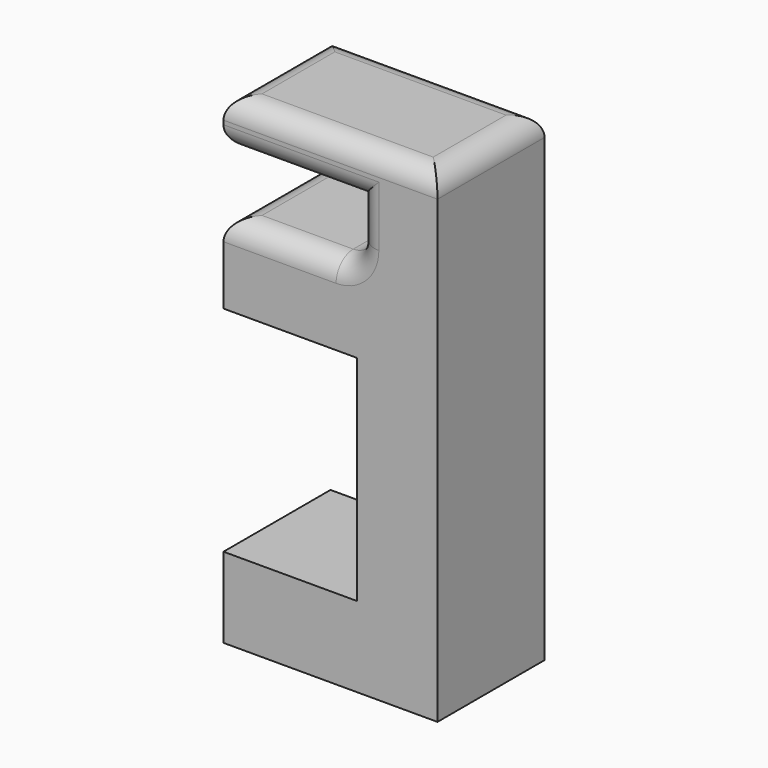
from build123d import *

# Parameters (mm, degrees)
F1_DEPTH = 5
F2_R     = 0.8


with BuildPart() as f1:
    # F0 (on Front) → F1 (new body)
    with BuildSketch(Plane.XZ):
        Polygon((0, 3), (0, 0), (8, 0), (8, 18), (0, 18), (0, 16.25), (5.0083114872, 16.25), (5.0083114872, 14), (0, 14), (0, 11), (5, 11), (5, 3), align=None)
    extrude(amount=F1_DEPTH)

    # F2
    f2_edges = [f1.edges().sort_by_distance(p)[0] for p in [
        (0, -2.5, 18),
        (0, -2.5, 16.25),
        (2.504156, -5, 14),
        (5.008311, -5, 15.125),
        (5.008311, 0, 15.125),
        (2.504156, -5, 16.25),
        (2.504156, 0, 14),
        (2.504156, 0, 16.25),
        (4, 0, 18),
        (4, -5, 18),
        (8, -2.5, 18),
        (5.008311, -2.5, 14),
        (0, -2.5, 14),
    ]]
    fillet(f2_edges, radius=F2_R)


solid = f1.part
